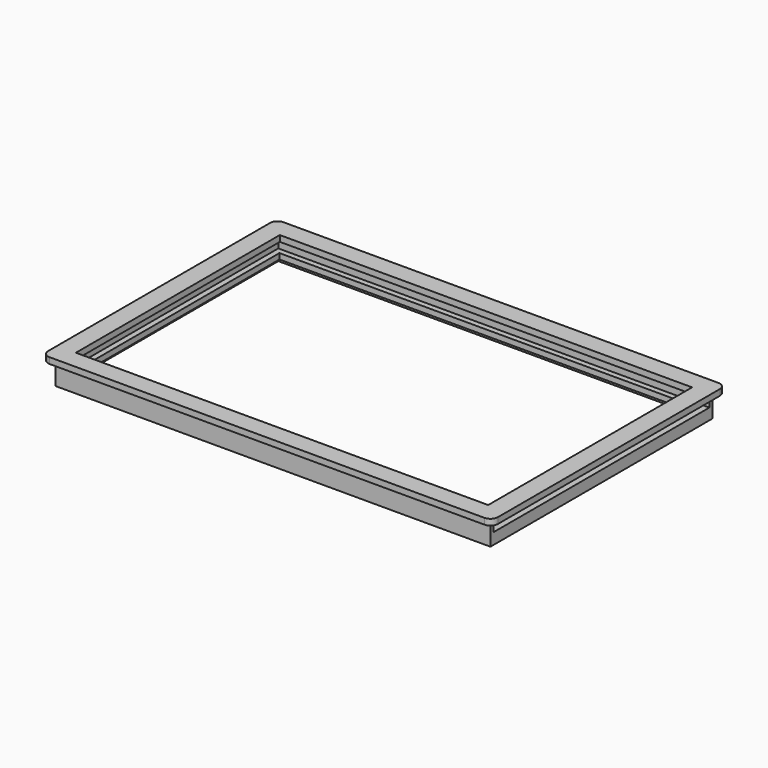
from build123d import *

# Parameters (mm, degrees)
F0_W     = 114
F0_H     = 72
F0_W_2   = 110
F0_H_2   = 68
F0_W_3   = 1
F1_DEPTH = 1.6
F2_DEPTH = 3
F3_W     = 114
F3_H     = 72
F3_W_2   = 111
F3_H_2   = 69
F4_DEPTH = 1.5
F5_DEPTH = 3
F3_W_3   = 1
F6_DEPTH = 3


with BuildPart() as f1:
    # F0 (on Top) → F1 (new body)
    with BuildSketch(Plane.XY):
        with BuildLine():
            Line((58, 39), (-58, 39))
            ThreePointArc((-58, 39), (-59.4142135624, 38.4142135624), (-60, 37))
            Line((-60, 37), (-60, -37))
            ThreePointArc((-60, -37), (-59.4142135624, -38.4142135624), (-58, -39))
            Line((-58, -39), (58, -39))
            ThreePointArc((58, -39), (59.4142135624, -38.4142135624), (60, -37))
            Line((60, -37), (60, 37))
            ThreePointArc((60, 37), (59.4142135624, 38.4142135624), (58, 39))
        make_face()
        Polygon((58, 37), (58, 36), (58, -36), (58, -37), (-58, -37), (-58, 37), align=None, mode=Mode.SUBTRACT)
        Polygon((-57, -36), (-57, 36), (57, 36), (58, 36), (58, 37), (-58, 37), (-58, -37), (58, -37), (58, -36), (57, -36), align=None)
        Rectangle(F0_W, F0_H)
        Rectangle(F0_W_2, F0_H_2, mode=Mode.SUBTRACT)
        with Locations((57.5, 0)):
            Rectangle(F0_W_3, F0_H)
    extrude(amount=F1_DEPTH)

    # F0 (on Top) → F2 (join)
    with BuildSketch(Plane.XY):
        Polygon((-57, -36), (-57, 36), (57, 36), (58, 36), (58, 37), (-58, 37), (-58, -37), (58, -37), (58, -36), (57, -36), align=None)
    extrude(amount=-F2_DEPTH)

    # F3 (on face) → F4 (join)
    with BuildSketch(Plane(origin=(0, 0, -3), x_dir=(1, 0, 0), z_dir=(0, 0, -1))):
        Rectangle(F3_W, F3_H)
        Rectangle(F3_W_2, F3_H_2, mode=Mode.SUBTRACT)
    extrude(amount=F4_DEPTH)

    # F5 (add): a face of the model
    f5_faces = [f1.faces().sort_by_distance(p)[0] for p in [
        (-57.1375936045, 0, -3),
    ]]
    extrude(f5_faces, amount=F5_DEPTH)

    # F3 (on face) → F6 (join)
    with BuildSketch(Plane(origin=(0, 0, -3), x_dir=(1, 0, 0), z_dir=(0, 0, -1))):
        with Locations((57.5, 0)):
            Rectangle(F3_W_3, F3_H)
    extrude(amount=F6_DEPTH)


solid = f1.part
